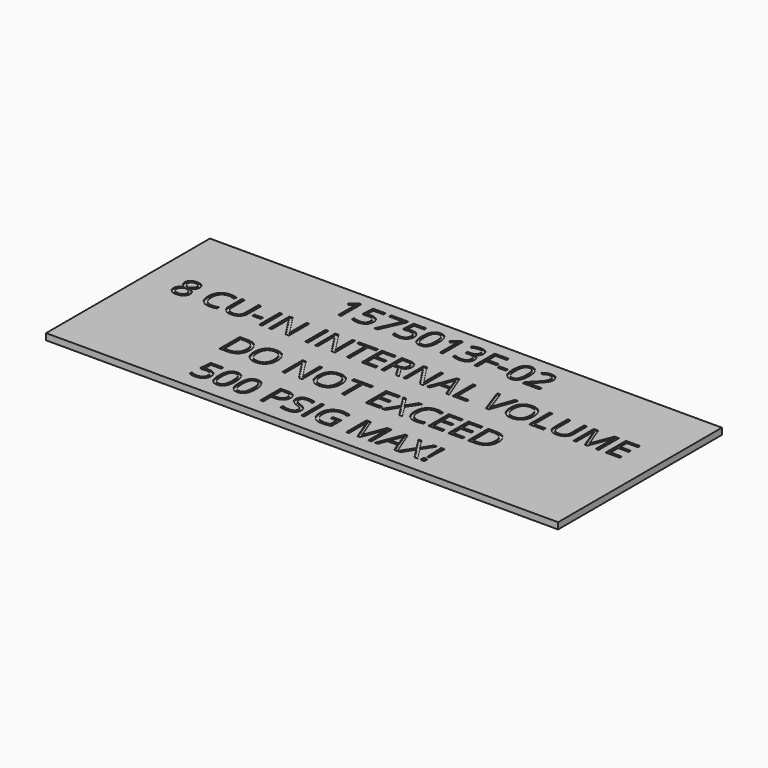
from build123d import *

# Parameters (mm, degrees)
F0_W         = 63.5
F0_H         = 25.4
F1_DEPTH     = 0.79375
F2_TEXT_SIZE = 4.4097222222
F3_DEPTH     = 0.127


# Not quite as in the source:
# - Text() gives the source's letters only with a copy of the font that has no kerning and outlines rounded to 1/6400 em; it was checked with that copy


with BuildPart() as f1:
    # F0 (on Top) → F1 (new body)
    with BuildSketch(Plane.XY):
        Rectangle(F0_W, F0_H)
    extrude(amount=F1_DEPTH)

    # F2 (on face) → F3 (cut)
    with BuildSketch(Plane.XY.offset(0.79375)):
        with Locations((-13.2171088325, 7.9375)):
            Text('1575013F-02', F2_TEXT_SIZE, font='Open Sans', text_align=(TextAlign.LEFT, TextAlign.BOTTOM))
        with Locations((-28.2556396484, 1.5875)):
            Text('8 CU-IN INTERNAL VOLUME', F2_TEXT_SIZE, font='Open Sans', text_align=(TextAlign.LEFT, TextAlign.BOTTOM))
        with Locations((-17.0273844401, -4.7625)):
            Text('DO NOT EXCEED', F2_TEXT_SIZE, font='Open Sans', text_align=(TextAlign.LEFT, TextAlign.BOTTOM))
        with Locations((-15.8815456814, -10.7597222222)):
            Text('500 PSIG MAX!', F2_TEXT_SIZE, font='Open Sans', text_align=(TextAlign.LEFT, TextAlign.BOTTOM))
    extrude(amount=-F3_DEPTH, mode=Mode.SUBTRACT)


solid = f1.part
